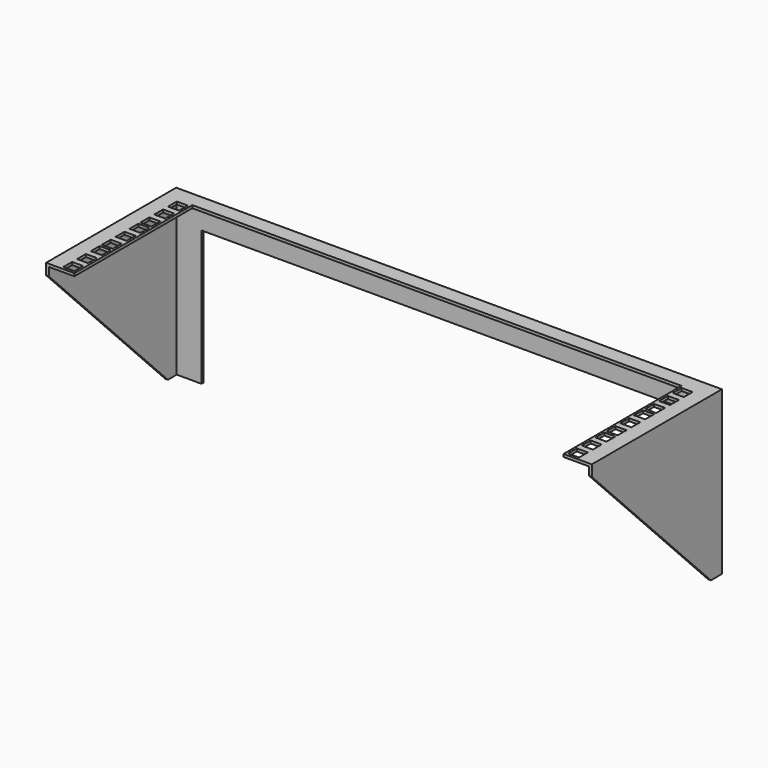
from build123d import *

# Parameters (mm, degrees)
F1_DEPTH = 2.54
F3_DEPTH = 2.54
F4_W     = 23.495
F4_H     = 147.32
F5_DEPTH = 2.54
F6_W     = 10.16
F6_H     = 10.16
F7_DEPTH = 25.4
F8_W     = 450.85
F8_H     = 11.43
F9_DEPTH = 2.54


# Not quite as in the source:
# - a pattern or mirror of a feature is missing from the dataset's text; its kind, count and spacing are read off the source's solid


with BuildPart() as f1:
    # F0 (on Front) → F1 (new body)
    with BuildSketch(Plane.XZ):
        Polygon((-226.06, -12.7), (226.06, -12.7), (226.06, -137.16), (251.46, -137.16), (251.46, -12.7), (251.46, 12.7), (-251.46, 12.7), (-251.46, -12.7), (-251.46, -137.16), (-226.06, -137.16), align=None)
    extrude(amount=F1_DEPTH)

    # F2 (on face) → F3 (join)
    with BuildSketch(Plane(origin=(-251.46, 0, 0), x_dir=(0, -1, 0), z_dir=(-1, 0, 0))):
        Polygon((149.86, 12.7), (2.54, 12.7), (2.54, -137.16), (12.7, -137.16), (149.86, 2.54), align=None)
    f3 = extrude(amount=-F3_DEPTH)

    # F3_copies: F3 across plane
    add(f3.mirror(Plane(origin=(0, 0, 0), x_dir=(0, 0, 1), z_dir=(1, 0, 0))))

    # F4 (on face) → F5 (join)
    with BuildSketch(Plane.XY.offset(12.7)):
        with Locations((-237.1725, -76.2)):
            Rectangle(F4_W, F4_H)
    f5 = extrude(amount=-F5_DEPTH)

    # F5_copies: F5 across plane
    add(f5.mirror(Plane(origin=(0, 0, 0), x_dir=(0, 0, 1), z_dir=(1, 0, 0))))

    # F6 (on face) → F7 (cut)
    with BuildSketch(Plane.XY.offset(12.7)):
        with Locations((-232.5624, -142.24)):
            Rectangle(F6_W, F6_H)
        with Locations((-232.5624, -126.365)):
            Rectangle(F6_W, F6_H)
        with Locations((-232.5624, -110.49)):
            Rectangle(F6_W, F6_H)
        with Locations((-232.5624, -97.79)):
            Rectangle(F6_W, F6_H)
        with Locations((-232.5624, -81.915)):
            Rectangle(F6_W, F6_H)
        with Locations((-232.5624, -66.04)):
            Rectangle(F6_W, F6_H)
        with Locations((-232.5624, -53.34)):
            Rectangle(F6_W, F6_H)
        with Locations((-232.5624, -37.465)):
            Rectangle(F6_W, F6_H)
        with Locations((-232.5624, -21.59)):
            Rectangle(F6_W, F6_H)
    f7 = extrude(amount=-F7_DEPTH, mode=Mode.SUBTRACT)

    # F7_copies: F7 across plane
    add(f7.mirror(Plane(origin=(0, 0, 0), x_dir=(0, 0, 1), z_dir=(1, 0, 0))), mode=Mode.SUBTRACT)

    # F8 (on face) → F9 (join)
    with BuildSketch(Plane.XY.offset(12.7)):
        with Locations((0, -8.255)):
            Rectangle(F8_W, F8_H)
    extrude(amount=-F9_DEPTH)


solid = f1.part
